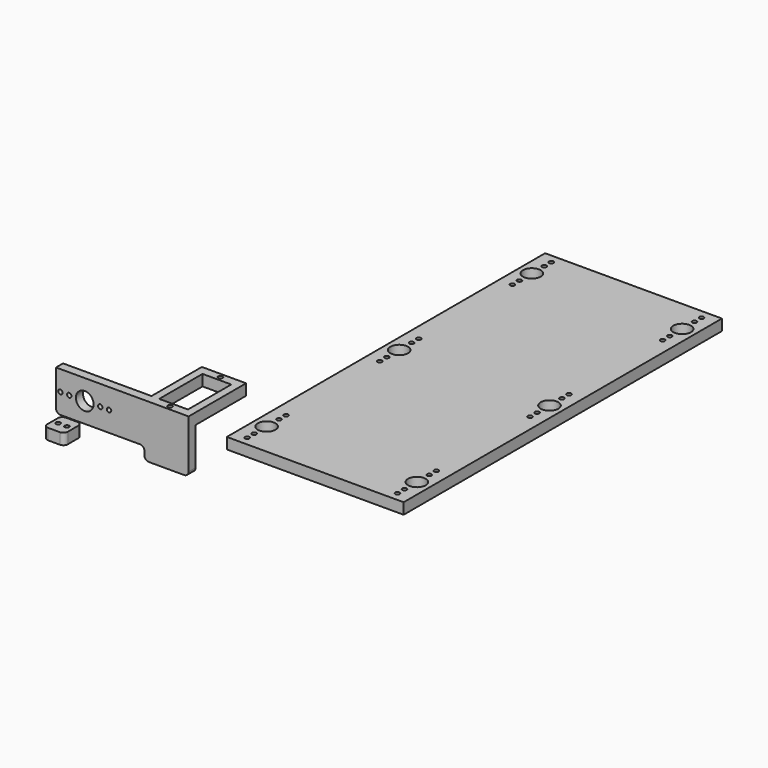
from build123d import *

# Parameters (mm, degrees)
F0_W     = 20
F0_H     = 32.5
F0_R     = 1
F0_W_2   = 13
F0_H_2   = 24.5
F1_DEPTH = 5
F2_R     = 1
F2_R_2   = 4
F3_DEPTH = 4
F4_R     = 2
F5_W     = 9.2630446101
F5_H     = 10
F5_R     = 1
F6_DEPTH = 5
F7_R     = 2
F8_W     = 80
F8_H     = 180
F8_R     = 1
F8_R_2   = 4
F9_DEPTH = 5


with BuildPart() as f1:
    # F0 (on Top) → F1 (new body)
    with BuildSketch(Plane.XY):
        with Locations((-30.3273589909, 20.0528247654)):
            Rectangle(F0_W, F0_H)
        with Locations((-30.3273589909, 5.8028247654)):
            Circle(F0_R, mode=Mode.SUBTRACT)
        with Locations((-30.3273589909, 20.0528247654)):
            Rectangle(F0_W_2, F0_H_2, mode=Mode.SUBTRACT)
        with Locations((-30.3273589909, 34.3028247654)):
            Circle(F0_R, mode=Mode.SUBTRACT)
    extrude(amount=F1_DEPTH)

    # F2 (on face) → F3 (join)
    with BuildSketch(Plane.XZ.offset(-3.8028247654)):
        Polygon((-20.3273589909, 0), (-40.3273589909, 0), (-40.3273589909, 5), (-80.3273589909, 5), (-80.3273589909, -13.25), (-40.3273589909, -13.25), (-40.3273589909, -19), (-20.3273589909, -19), align=None)
        with Locations((-78.3273589909, -4.125)):
            Circle(F2_R, mode=Mode.SUBTRACT)
        with Locations((-74.3273589909, -4.125)):
            Circle(F2_R, mode=Mode.SUBTRACT)
        with Locations((-67.3273589909, -4.125)):
            Circle(F2_R_2, mode=Mode.SUBTRACT)
        with Locations((-60.3273589909, -4.125)):
            Circle(F2_R, mode=Mode.SUBTRACT)
        with Locations((-56.3273589909, -4.125)):
            Circle(F2_R, mode=Mode.SUBTRACT)
    extrude(amount=-F3_DEPTH)

    # F4
    f4_edges = [f1.edges().sort_by_distance(p)[0] for p in [
        (-40.327359, 5.802825, -13.25),
        (-40.327359, 5.802825, -19),
        (-20.327359, 5.802825, -19),
        (-80.327359, 5.802825, -13.25),
    ]]
    fillet(f4_edges, radius=F4_R)


with BuildPart() as f6:
    # F5 (on Top) → F6 (new body)
    with BuildSketch(Plane.XY):
        with Locations((-50.9674716741, -29.0176426284)):
            Rectangle(F5_W, F5_H)
        with Locations((-53.0989939792, -29.0176426284)):
            Circle(F5_R, mode=Mode.SUBTRACT)
        with Locations((-49.0989939792, -29.0176426284)):
            Circle(F5_R, mode=Mode.SUBTRACT)
    extrude(amount=F6_DEPTH)

    # F7
    f7_edges = [f6.edges().sort_by_distance(p)[0] for p in [
        (-55.598994, -24.017643, 2.5),
        (-46.335949, -24.017643, 2.5),
        (-55.598994, -34.017643, 2.5),
        (-46.335949, -34.017643, 2.5),
    ]]
    fillet(f7_edges, radius=F7_R)


with BuildPart() as f9:
    # F8 (on Top) → F9 (new body)
    with BuildSketch(Plane.XY):
        with Locations((40, 90)):
            Rectangle(F8_W, F8_H)
        with Locations((6, 4)):
            Circle(F8_R, mode=Mode.SUBTRACT)
        with Locations((6, 8)):
            Circle(F8_R, mode=Mode.SUBTRACT)
        with Locations((6, 15)):
            Circle(F8_R_2, mode=Mode.SUBTRACT)
        with Locations((6, 22)):
            Circle(F8_R, mode=Mode.SUBTRACT)
        with Locations((6, 26)):
            Circle(F8_R, mode=Mode.SUBTRACT)
        with Locations((6, 79)):
            Circle(F8_R, mode=Mode.SUBTRACT)
        with Locations((6, 83)):
            Circle(F8_R, mode=Mode.SUBTRACT)
        with Locations((74, 4)):
            Circle(F8_R, mode=Mode.SUBTRACT)
        with Locations((74, 8)):
            Circle(F8_R, mode=Mode.SUBTRACT)
        with Locations((74, 15)):
            Circle(F8_R_2, mode=Mode.SUBTRACT)
        with Locations((74, 22)):
            Circle(F8_R, mode=Mode.SUBTRACT)
        with Locations((74, 26)):
            Circle(F8_R, mode=Mode.SUBTRACT)
        with Locations((74, 79)):
            Circle(F8_R, mode=Mode.SUBTRACT)
        with Locations((74, 83)):
            Circle(F8_R, mode=Mode.SUBTRACT)
        with Locations((6, 90)):
            Circle(F8_R_2, mode=Mode.SUBTRACT)
        with Locations((6, 97)):
            Circle(F8_R, mode=Mode.SUBTRACT)
        with Locations((6, 101)):
            Circle(F8_R, mode=Mode.SUBTRACT)
        with Locations((6, 154)):
            Circle(F8_R, mode=Mode.SUBTRACT)
        with Locations((6, 158)):
            Circle(F8_R, mode=Mode.SUBTRACT)
        with Locations((6, 165)):
            Circle(F8_R_2, mode=Mode.SUBTRACT)
        with Locations((6, 172)):
            Circle(F8_R, mode=Mode.SUBTRACT)
        with Locations((6, 176)):
            Circle(F8_R, mode=Mode.SUBTRACT)
        with Locations((74, 90)):
            Circle(F8_R_2, mode=Mode.SUBTRACT)
        with Locations((74, 97)):
            Circle(F8_R, mode=Mode.SUBTRACT)
        with Locations((74, 101)):
            Circle(F8_R, mode=Mode.SUBTRACT)
        with Locations((74, 154)):
            Circle(F8_R, mode=Mode.SUBTRACT)
        with Locations((74, 158)):
            Circle(F8_R, mode=Mode.SUBTRACT)
        with Locations((74, 165)):
            Circle(F8_R_2, mode=Mode.SUBTRACT)
        with Locations((74, 172)):
            Circle(F8_R, mode=Mode.SUBTRACT)
        with Locations((74, 176)):
            Circle(F8_R, mode=Mode.SUBTRACT)
    extrude(amount=F9_DEPTH)


solid = Compound([f1.part, f6.part, f9.part])
